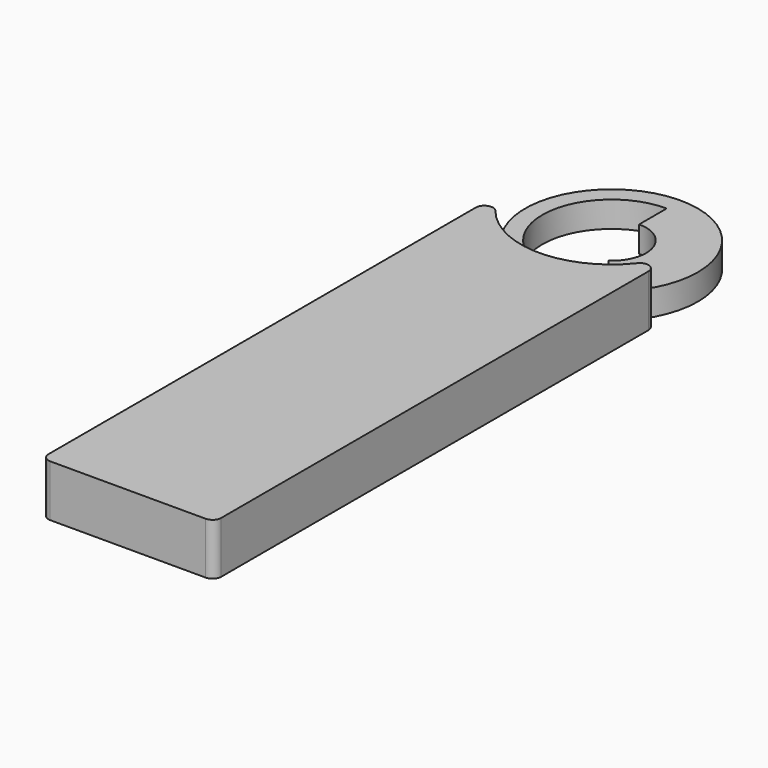
from build123d import *

# Parameters (mm, degrees)
F1_DEPTH = 6
F2_DEPTH = 3
F3_R     = 1


with BuildPart() as f1:
    # F0 (on Top) → F1 (new body)
    with BuildSketch(Plane.XY):
        with BuildLine():
            Line((10, -70), (10, -3.2015621187))
            ThreePointArc((10, -3.2015621187), (0, -10.5), (-10, -3.2015621187))
            Line((-10, -3.2015621187), (-10, -70))
            Line((-10, -70), (10, -70))
        make_face()
    extrude(amount=F1_DEPTH)

    # F3
    f3_edges = [f1.edges().sort_by_distance(p)[0] for p in [
        (10, -70, 3),
        (-10, -70, 3),
        (10, -3.201562, 3),
        (-10, -3.201562, 3),
    ]]
    fillet(f3_edges, radius=F3_R)


with BuildPart() as f2:
    # F0 (on Top) → F2 (new body)
    with BuildSketch(Plane.XY):
        with BuildLine():
            ThreePointArc((-10, 0), (0, -10), (10, 0))
            ThreePointArc((10, 0), (0, 10), (-10, 0))
        make_face()
        with BuildLine():
            ThreePointArc((0, 8), (5.6568542495, 5.6568542495), (8, 0))
            ThreePointArc((8, 0), (7.0960866654, -3.6939889059), (4.5886114908, -6.5532163543))
            ThreePointArc((4.5886114908, -6.5532163543), (0, -8), (-4.5886114908, -6.5532163543))
            ThreePointArc((-4.5886114908, -6.5532163543), (-7.629735606, 2.405646396), (0, 8))
        make_face(mode=Mode.SUBTRACT)
        with BuildLine():
            ThreePointArc((4.5886114908, -6.5532163543), (7.0960866654, -3.6939889059), (8, 0))
            ThreePointArc((8, 0), (5.6568542495, 5.6568542495), (0, 8))
            Line((0, 8), (0, 4))
            ThreePointArc((0, 4), (2.8284271247, 2.8284271247), (4, 0))
            ThreePointArc((4, 0), (3.5480433327, -1.8469944529), (2.2943057454, -3.2766081772))
            Line((2.2943057454, -3.2766081772), (4.5886114908, -6.5532163543))
        make_face()
    extrude(amount=F2_DEPTH)


solid = Compound([f1.part, f2.part])
